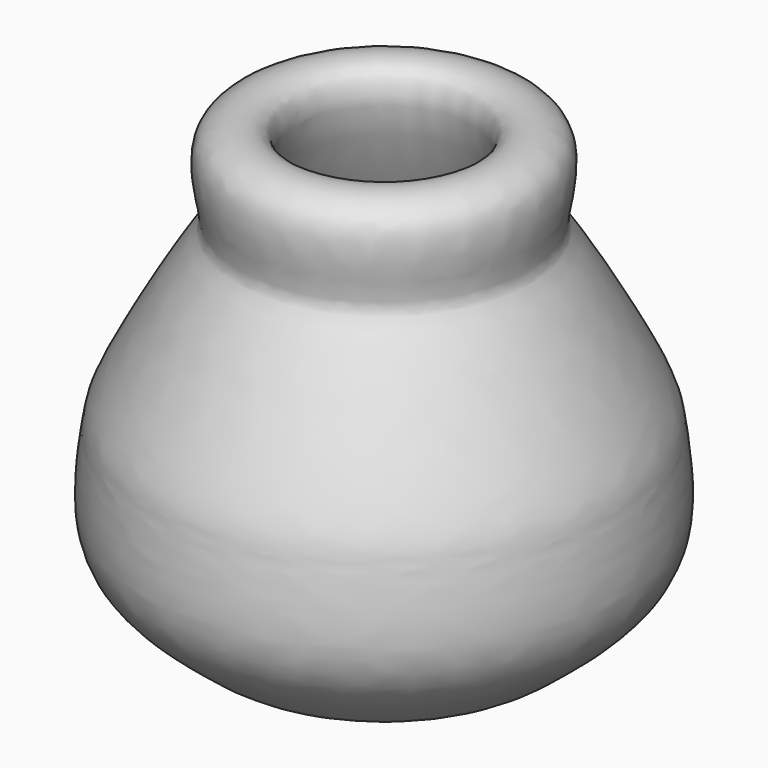
from build123d import *


with BuildPart() as f1:
    # F0 (on Front) → F1 (revolve)
    with BuildSketch(Plane.XZ):
        with BuildLine():
            add(Edge.make_bspline(
                [(-25.6102147929, 61.8484951556), (-19.4896790224, 49.6324052715), (-66.2156119978, -18.1700595461), (-52.5415644786, -39.3807960779), (-30.8517184463, -55.2794042637), (-18.0136531138, -51.3594918991), (-11.6013032839, -59.8924308511), (-11.5742936307, -66.8086153132), (-21.3751043638, -69.4109851577), (-42.7577735512, -65.6699253484), (-50.7702194774, -58.671854983), (-68.5979939867, -44.7055573728), (-69.8158166263, -26.367830304), (-67.5266448655, -11.3340150059), (-66.384422734, -3.2803288068), (-44.9160500553, 34.4068090372), (-39.389543016, 39.7040882329), (-48.5030660848, 65.5862712276), (-28.244051641, 67.1054185497), (-25.6102147929, 61.8484951556)],
                knots=[0, 0, 0, 0, 0.1274952524, 0.1945854023, 0.2631051441, 0.3103880092, 0.351834689, 0.3840898167, 0.4248217112, 0.4886012713, 0.5353180464, 0.598755054, 0.6577011126, 0.7095539001, 0.7519960135, 0.8414283616, 0.8822145077, 0.9451352453, 1, 1, 1, 1], degree=3))
        make_face()
    revolve(axis=Axis((0, 0, -13.5012418032), (0, 0, -1)))


solid = f1.part
